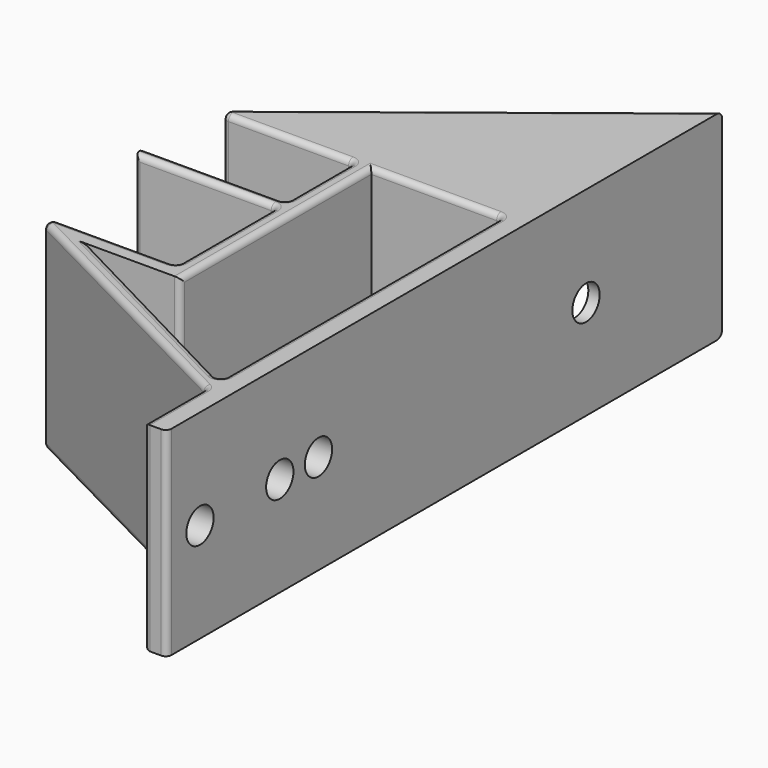
from build123d import *

# Parameters (mm, degrees)
F1_DEPTH    = 35
F3_T        = 2
F3_T3_DEPTH = 39
F4_R        = 3
F5_DEPTH    = 25
F6_R        = 3
F7_DEPTH    = 5.9
F8_R        = 0.99999
F9_R        = 3
F10_DEPTH   = 25
F11_R       = 3
F12_DEPTH   = 25


# Not quite as in the source:
# - a fillet or chamfer is up to 0.001 mm smaller than in the source, because OpenCascade refuses the exact size
# - a shell that OpenCascade refuses in one call is made with other operations: the cavity is built on its own and cut out
# - a feature names something its author has since deleted; it is built from what else it names


with BuildPart() as f1:
    # F0 (on Top) → F1 (new body)
    with BuildSketch(Plane.XY):
        Polygon((0, -35.5268927627), (-25, -35.5268927627), (26, -61.7087109445), (26, -75.1632548192), (30, -75.1632548192), (30, 43.5640147483), (30, 46.7083996511), (26, 43.5640147483), (-25, 3.4731072373), (0, 3.4731072373), (0, -11.5268927627), (-25, -11.5268927627), (-25, -13.5268927627), (0, -13.5268927627), align=None)
        Polygon((3, -38.5268927627), (3, 3.4731072373), (26, 3.4731072373), (26, -58.7087109445), (-12.7289108932, -38.5268927627), align=None, mode=Mode.SUBTRACT)
    extrude(amount=F1_DEPTH)

    # F3: shell of thickness 2, made by hand


with BuildPart() as f3_core1:
    # F3_t2: copy of F1
    add(f1.part)

    # the walls: a layer under each face that stays
    f3_faces = [f3_core1.faces().sort_by_distance(p)[0] for p in [
        (-12.5, 3.4731072373, 17.5),
        (2.5, -14.227427584, 35),
        (-4.8644554466, -38.5268927627, 17.5),
        (6.6355445534, -48.6178018536, 17.5),
        (26, -27.6178018536, 17.5),
        (14.5, 3.4731072373, 17.5),
        (3, -17.5268927627, 17.5),
        (30, -14.227427584, 17.5),
        (28, -75.1632548192, 17.5),
        (26, -68.4359828818, 17.5),
        (0.5, -48.6178018536, 17.5),
        (-12.5, -35.5268927627, 17.5),
        (0, -24.5268927627, 17.5),
        (-12.5, -13.5268927627, 17.5),
        (-25, -12.5268927627, 17.5),
        (-12.5, -11.5268927627, 17.5),
        (2.5, -14.227427584, 0),
        (0, -4.0268927627, 17.5),
    ]]
    thicken(f3_faces, amount=-F3_T, mode=Mode.SUBTRACT)

    # F3_s4 → F3_t3 (cut)
    with BuildSketch(Plane.XY.offset(-2)):
        Polygon((-0.02, 3.4531072373), (0, 5.4731072373), (2, 5.4731072373), (2, 3.4731072373), align=None)
        Polygon((-12.7196684188, -38.5291564534), (-12.7289108932, -36.5268927627), (-20.8947564215, -36.5268927627), (-13.6531583366, -40.3005236892), align=None)
        Polygon((25.9892424744, -58.6909746353), (25.0757525566, -60.482341871), (28, -62.0061810098), (28, -58.7087109445), align=None)
        Polygon((25.98, 3.4531072373), (28, 3.4731072373), (28, 5.4731072373), (26, 5.4731072373), align=None)
        Polygon((3.02, 3.4531072373), (3, 5.4731072373), (1, 5.4731072373), (1, 3.4731072373), align=None)
        Polygon((25.9708659413, -61.7265033297), (28, -61.7087109445), (28, -60.4872961474), (26.9134058716, -59.9294724238), align=None)
        Polygon((-0.02, -35.5068927627), (0, -37.5268927627), (2, -37.5268927627), (2, -35.5268927627), align=None)
        Polygon((-0.02, -13.5468927627), (2, -13.5268927627), (2, -11.5268927627), (0, -11.5268927627), align=None)
        Polygon((-0.02, -11.5068927627), (0, -13.5268927627), (2, -13.5268927627), (2, -11.5268927627), align=None)
    extrude(amount=F3_T3_DEPTH, mode=Mode.SUBTRACT)


with BuildPart() as f1_1:
    add(f1.part)

    # what is left inside the walls is the cavity
    f3_cavity = [f3_core1.part.solids().sort_by_distance(p)[0] for p in [
        (2.784469, 25.288934, 22.666667),
    ]]
    add(f3_cavity, mode=Mode.SUBTRACT)

    # F4 (on face) → F5 (cut)
    with BuildSketch(Plane(origin=(28, 0, 0), x_dir=(0, -1, 0), z_dir=(-1, 0, 0))):
        with Locations((-16.8671440333, 17.5)):
            Circle(F4_R)
    extrude(amount=-F5_DEPTH, mode=Mode.SUBTRACT)

    # F6 (on face) → F7 (cut)
    with BuildSketch(Plane(origin=(0, 5.4731072373, 0), x_dir=(-1, 0, 0), z_dir=(0, 1, 0))):
        with Locations((13.21292707, 17.5)):
            Circle(F6_R)
    extrude(amount=-F7_DEPTH, mode=Mode.SUBTRACT)

    # F8 (radius 1 in the source; OpenCascade refuses exactly that, so slightly less here)
    f8_edges = [f1_1.edges().sort_by_distance(p)[0] for p in [
        (2.5, 25.090753, 35),
        (2.5, 25.090753, 0),
        (-25, 3.473107, 17.5),
        (-12.5, 3.473107, 35),
        (-12.5, 3.473107, 0),
        (0, 3.473107, 17.5),
        (0, -11.526893, 17.5),
        (0, -13.526893, 17.5),
        (-25, -13.526893, 17.5),
        (-12.5, -13.526893, 0),
        (-12.5, -13.526893, 35),
        (-25, -11.526893, 17.5),
        (0, -35.526893, 17.5),
        (-25, -35.526893, 17.5),
        (0.5, -48.617802, 35),
        (0.5, -48.617802, 0),
        (26, -61.708711, 17.5),
        (3, -17.526893, 35),
        (6.635545, -48.617802, 35),
        (26, -27.617802, 35),
        (14.5, 3.473107, 35),
        (3, -17.526893, 0),
        (14.5, 3.473107, 0),
        (26, -27.617802, 0),
        (6.635545, -48.617802, 0),
        (26, -75.163255, 17.5),
        (3, -38.526893, 17.5),
        (26, -58.708711, 17.5),
        (26, 3.473107, 17.5),
        (2.772109, 25.304657, 33),
        (2.772109, 25.304657, 2),
        (0, -4.026893, 0),
        (-12.5, -11.526893, 0),
        (0, -24.526893, 0),
        (-12.5, -35.526893, 0),
        (26, -68.435983, 0),
        (0, -4.026893, 35),
        (-12.5, -11.526893, 35),
        (0, -24.526893, 35),
        (-12.5, -35.526893, 35),
        (26, -68.435983, 35),
        (30, -75.163255, 17.5),
        (28, 5.473107, 17.5),
    ]]
    fillet(f8_edges, radius=F8_R)

    # F9 (on face) → F10 (cut)
    with BuildSketch(Plane(origin=(26, 0, 0), x_dir=(0, -1, 0), z_dir=(-1, 0, 0))):
        with Locations((50.3810942173, 17.5)):
            Circle(F9_R)
        with Locations((41.8810732663, 17.5000000745)):
            Circle(F9_R)
    extrude(amount=-F10_DEPTH, mode=Mode.SUBTRACT)

    # F11 (on face) → F12 (cut)
    with BuildSketch(Plane(origin=(26, 0, 0), x_dir=(0, -1, 0), z_dir=(-1, 0, 0))):
        with Locations((67.9058432579, 17.5)):
            Circle(F11_R)
    extrude(amount=-F12_DEPTH, mode=Mode.SUBTRACT)


solid = f1_1.part
